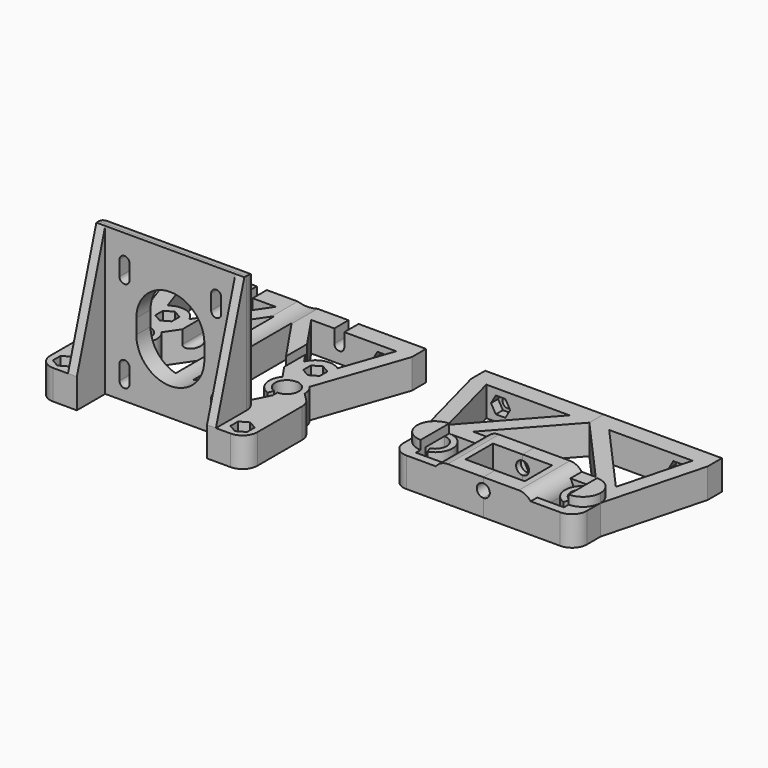
from build123d import *
from build123d import SkipClean  # not in build123d's __all__

# Parameters (mm, degrees)
F1_DEPTH  = 10
F0_R      = 1.7
F2_DEPTH  = 3
F3_DEPTH  = 50
F4_W      = 3.4
F4_H      = 5
F5_DEPTH  = 58.001
F7_DEPTH  = 5
F8_R      = 1.75
F9_DEPTH  = 8
F10_DEPTH = 3
F11_R     = 5
F13_DEPTH = 13
F14_DEPTH = 10
F15_DEPTH = 10
F16_DEPTH = 12
F18_DEPTH = 40.801
F19_DEPTH = 3
F20_R     = 1.75
F21_DEPTH = 10
F22_DEPTH = 3
F23_R     = 5


with BuildPart() as f1:
    # F0 (on Top) → F1 (new body)
    with BuildSketch(Plane.XY):
        with BuildLine():
            Line((40, 0), (0, 0))
            Line((0, 0), (0, -52))
            Line((0, -52), (3, -52))
            Line((3, -52), (3, -10.4836443767))
            Line((3, -10.4836443767), (20.4082464152, -36.1379022518))
            ThreePointArc((20.4082464152, -36.1379022518), (24.9775015641, -34.0000421818), (29.5626609437, -36.1035753424))
            Line((29.5626609437, -36.1035753424), (40, -6))
            Line((40, -6), (40, 0))
        make_face()
        Polygon((25, -24.7668384925), (27.8, -26.3834192463), (27.8, -29.6165807537), (25, -31.2331615075), (22.2, -29.6165807537), (22.2, -26.3834192463), align=None, mode=Mode.SUBTRACT)
        with BuildLine():
            Line((6, -6), (34.7079994735, -6))
            Line((34.7079994735, -6), (28.7140967276, -23.2877303242))
            ThreePointArc((28.7140967276, -23.2877303242), (23.4432894869, -22.2054635752), (19.4244541485, -25.7834061135))
            Line((19.4244541485, -25.7834061135), (6, -6))
        make_face(mode=Mode.SUBTRACT)
        with BuildLine():
            ThreePointArc((31, -40), (30.629208011, -37.9234602896), (29.5626609437, -36.1035753424))
            ThreePointArc((29.5626609437, -36.1035753424), (24.9775015641, -34.0000421818), (20.4082464152, -36.1379022518))
            ThreePointArc((20.4082464152, -36.1379022518), (19.2107499955, -41.5762564467), (23, -45.6568542495))
            Line((23, -45.6568542495), (23.6666666667, -43.7712361663))
            ThreePointArc((23.6666666667, -43.7712361663), (22.6905989232, -36.7340136763), (29, -40))
            ThreePointArc((29, -40), (27.8284271247, -42.8284271247), (25, -44))
            Line((25, -44), (25, -46))
            ThreePointArc((25, -46), (29.2426406871, -44.2426406871), (31, -40))
        make_face()
        Polygon((22, -52), (22, -58), (22, -70), (25, -70), (25, -52), align=None)
        Polygon((3, -52), (0, -52), (0, -58), (22, -58), (22, -52), align=None)
        with BuildLine():
            Line((35, -44), (31, -40))
            ThreePointArc((31, -40), (29.2426406871, -44.2426406871), (25, -46))
            Line((25, -46), (25, -52))
            Line((25, -52), (25, -70))
            Line((25, -70), (35, -70))
            Line((35, -70), (35, -44))
        make_face()
        Polygon((30, -61.7668384925), (32.8, -63.3834192463), (32.8, -66.6165807537), (30, -68.2331615075), (27.2, -66.6165807537), (27.2, -63.3834192463), align=None, mode=Mode.SUBTRACT)
        Polygon((25, -46), (22, -52), (25, -52), align=None)
    extrude(amount=F1_DEPTH)

    # F0 (on Top) → F2 (join)
    with BuildSketch(Plane.XY):
        Polygon((27.8, -29.6165807537), (27.8, -26.3834192463), (25, -24.7668384925), (22.2, -26.3834192463), (22.2, -29.6165807537), (25, -31.2331615075), align=None)
        with Locations((25, -28)):
            Circle(F0_R, mode=Mode.SUBTRACT)
        Polygon((32.8, -66.6165807537), (32.8, -63.3834192463), (30, -61.7668384925), (27.2, -63.3834192463), (27.2, -66.6165807537), (30, -68.2331615075), align=None)
        with Locations((30, -65)):
            Circle(F0_R, mode=Mode.SUBTRACT)
    extrude(amount=F2_DEPTH)

    # F0 (on Top) → F3 (join)
    with BuildSketch(Plane.XY):
        Polygon((3, -52), (0, -52), (0, -58), (22, -58), (22, -52), align=None)
        Polygon((22, -52), (22, -58), (22, -70), (25, -70), (25, -52), align=None)
    extrude(amount=F3_DEPTH)

    # F4 (on face) → F5 (cut, through all)
    with BuildSketch(Plane.XZ.offset(58)):
        with BuildLine():
            ThreePointArc((17.2, 10.5), (15.5, 12.2), (13.8, 10.5))
            Line((13.8, 10.5), (17.2, 10.5))
        make_face()
        with Locations((15.5, 8)):
            Rectangle(F4_W, F4_H)
        with BuildLine():
            Line((17.2, 5.5), (13.8, 5.5))
            ThreePointArc((13.8, 5.5), (15.5, 3.8), (17.2, 5.5))
        make_face()
        with BuildLine():
            Line((13.8, 41.5), (13.8, 36.5))
            ThreePointArc((13.8, 36.5), (15.5, 34.8), (17.2, 36.5))
            Line((17.2, 36.5), (17.2, 41.5))
            ThreePointArc((17.2, 41.5), (15.5, 43.2), (13.8, 41.5))
        make_face()
        with BuildLine():
            Line((11.5, 21), (11.5, 26))
            ThreePointArc((11.5, 26), (0, 37.5), (-11.5, 26))
            Line((-11.5, 26), (-11.5, 21))
            ThreePointArc((-11.5, 21), (0, 9.5), (11.5, 21))
        make_face()
    extrude(amount=-F5_DEPTH, mode=Mode.SUBTRACT)

    # F6 (on face) → F7 (cut)
    with BuildSketch(Plane.YZ.offset(25)):
        Polygon((-70, 10), (-58, 50), (-70, 50), align=None)
    extrude(amount=-F7_DEPTH, mode=Mode.SUBTRACT)

    # F8 (on face) → F9 (cut)
    with BuildSketch(Plane(origin=(0, 0, 0), x_dir=(-1, 0, 0), z_dir=(0, 1, 0))):
        Polygon((-28.3834192463, 7.8), (-31.6165807537, 7.8), (-33.2331615075, 5), (-31.6165807537, 2.2), (-28.3834192463, 2.2), (-26.7668384925, 5), align=None)
        with Locations((-30, 5)):
            Circle(F8_R, mode=Mode.SUBTRACT)
        with Locations((-30, 5)):
            Circle(F8_R)
    extrude(amount=-F9_DEPTH, mode=Mode.SUBTRACT)

    # F8 (on face) → F10 (join)
    with BuildSketch(Plane(origin=(0, 0, 0), x_dir=(-1, 0, 0), z_dir=(0, 1, 0))):
        Polygon((-28.3834192463, 7.8), (-31.6165807537, 7.8), (-33.2331615075, 5), (-31.6165807537, 2.2), (-28.3834192463, 2.2), (-26.7668384925, 5), align=None)
        with Locations((-30, 5)):
            Circle(F8_R, mode=Mode.SUBTRACT)
    extrude(amount=-F10_DEPTH)

    # F11
    f11_edges = [f1.edges().sort_by_distance(p)[0] for p in [
        (12.5, -52, 50),
        (25, -52, 30),
        (35, -44, 5),
        (35, -70, 5),
    ]]
    fillet(f11_edges, radius=F11_R)

    # F12: F1 across plane


with BuildPart() as f1_1:
    add(f1.part, clean=False)
    add(f1.part.mirror(Plane.YZ), clean=False)


with BuildPart() as f13:
    # F0 (on Top) → F13 (new body)
    with BuildSketch(Plane.XY):
        with BuildLine():
            ThreePointArc((131, -40), (129.2426406871, -35.7573593129), (125, -34))
            Line((125, -34), (125, -36))
            ThreePointArc((125, -36), (127.8284271247, -37.1715728753), (129, -40))
            ThreePointArc((129, -40), (127.8284271247, -42.8284271247), (125, -44))
            Line((125, -44), (125, -46))
            ThreePointArc((125, -46), (129.2426406871, -44.2426406871), (131, -40))
        make_face()
        with BuildLine():
            ThreePointArc((129, -40), (127.8284271247, -37.1715728753), (125, -36))
            Line((125, -36), (125, -40))
            Line((125, -40), (125, -44))
            ThreePointArc((125, -44), (127.8284271247, -42.8284271247), (129, -40))
        make_face()
    extrude(amount=F13_DEPTH)

    # F0 (on Top) → F14 (cut)
    with BuildSketch(Plane.XY):
        with BuildLine():
            ThreePointArc((129, -40), (127.8284271247, -37.1715728753), (125, -36))
            Line((125, -36), (125, -40))
            Line((125, -40), (125, -44))
            ThreePointArc((125, -44), (127.8284271247, -42.8284271247), (129, -40))
        make_face()
    extrude(amount=F14_DEPTH, mode=Mode.SUBTRACT)

    # F0 (on Top) → F15 (join)
    with BuildSketch(Plane.XY):
        with BuildLine():
            Line((106.7029729925, -6), (100, -6))
            Line((100, -6), (120.7142857143, -29.2))
            Line((120.7142857143, -29.2), (125, -34))
            ThreePointArc((125, -34), (129.2426406871, -35.7573593129), (131, -40))
            Line((131, -40), (140, -6))
            Line((140, -6), (134.8277925309, -6))
            Line((134.8277925309, -6), (128.3963455947, -30.2965773144))
            Line((128.3963455947, -30.2965773144), (106.7029729925, -6))
        make_face()
        Polygon((125, -34), (120.7142857143, -29.2), (117, -29.2), (117, -34), align=None)
        with BuildLine():
            Line((125, -36), (125, -34))
            ThreePointArc((125, -34), (119.0864086421, -38.9853881276), (123, -45.6568542495))
            Line((123, -45.6568542495), (123.6666666667, -43.7712361663))
            ThreePointArc((123.6666666667, -43.7712361663), (121.0576057614, -39.3235920851), (125, -36))
        make_face()
        with BuildLine():
            Line((131, -50.8), (131, -40))
            ThreePointArc((131, -40), (129.2426406871, -44.2426406871), (125, -46))
            Line((125, -46), (125, -48))
            Line((125, -48), (117, -48))
            Line((117, -48), (117, -50.8))
            Line((117, -50.8), (131, -50.8))
        make_face()
        Polygon((140, 0), (100, 0), (100, -6), (106.7029729925, -6), (134.8277925309, -6), (140, -6), align=None)
    extrude(amount=F15_DEPTH)

    # F0 (on Top) → F16 (join)
    with BuildSketch(Plane.XY):
        Polygon((117, -34), (117, -29.2), (100, -29.2), (100, -34.2), (110, -34.2), (110, -45.8), (100, -45.8), (100, -50.8), (117, -50.8), (117, -48), align=None)
    extrude(amount=F16_DEPTH)

    # F17 (on face) → F18 (cut, through all)
    with BuildSketch(Plane(origin=(0, -29.2, 0), x_dir=(-1, 0, 0), z_dir=(0, 1, 0))):
        with BuildLine():
            Line((-100, 5.8), (-100, 10.2))
            ThreePointArc((-100, 10.2), (-102.2, 8), (-100, 5.8))
        make_face()
    extrude(amount=-F18_DEPTH, mode=Mode.SUBTRACT)

    # F17 (on face) → F19 (cut)
    with BuildSketch(Plane(origin=(0, -29.2, 0), x_dir=(-1, 0, 0), z_dir=(0, 1, 0))):
        with BuildLine():
            ThreePointArc((-100, 5.8), (-102.2, 8), (-100, 10.2))
            Line((-100, 10.2), (-100, 11.65))
            Line((-100, 11.65), (-102.1073284825, 11.65))
            Line((-102.1073284825, 11.65), (-104.2146569651, 8))
            Line((-104.2146569651, 8), (-102.1073284825, 4.35))
            Line((-102.1073284825, 4.35), (-100, 4.35))
            Line((-100, 4.35), (-100, 5.8))
        make_face()
    extrude(amount=-F19_DEPTH, mode=Mode.SUBTRACT)

    # F20 (on face) → F21 (cut)
    with BuildSketch(Plane(origin=(0, 0, 0), x_dir=(-1, 0, 0), z_dir=(0, 1, 0))):
        Polygon((-128.3834192463, 7.8), (-131.6165807537, 7.8), (-133.2331615075, 5), (-131.6165807537, 2.2), (-128.3834192463, 2.2), (-126.7668384925, 5), align=None)
        with Locations((-130, 5)):
            Circle(F20_R, mode=Mode.SUBTRACT)
        with Locations((-130, 5)):
            Circle(F20_R)
    extrude(amount=-F21_DEPTH, mode=Mode.SUBTRACT)

    # F20 (on face) → F22 (join)
    with BuildSketch(Plane(origin=(0, 0, 0), x_dir=(-1, 0, 0), z_dir=(0, 1, 0))):
        Polygon((-128.3834192463, 7.8), (-131.6165807537, 7.8), (-133.2331615075, 5), (-131.6165807537, 2.2), (-128.3834192463, 2.2), (-126.7668384925, 5), align=None)
        with Locations((-130, 5)):
            Circle(F20_R, mode=Mode.SUBTRACT)
    extrude(amount=-F22_DEPTH)

    # F23
    f23_edges = [f13.edges().sort_by_distance(p)[0] for p in [
        (131, -50.8, 5),
        (117, -40, 12),
    ]]
    fillet(f23_edges, radius=F23_R)

    # F24: F13 across face


with BuildPart() as f13_1:
    add(f13.part, clean=False)
    with SkipClean():  # cleaning this boolean's faces spoils the solid; the shape is the same uncleaned
        add(f13.part.mirror(Plane(origin=(100, -3, 5), x_dir=(0, -1, 0), z_dir=(-1, 0, 0))), clean=False)


solid = Compound([f1_1.part, f13_1.part])
